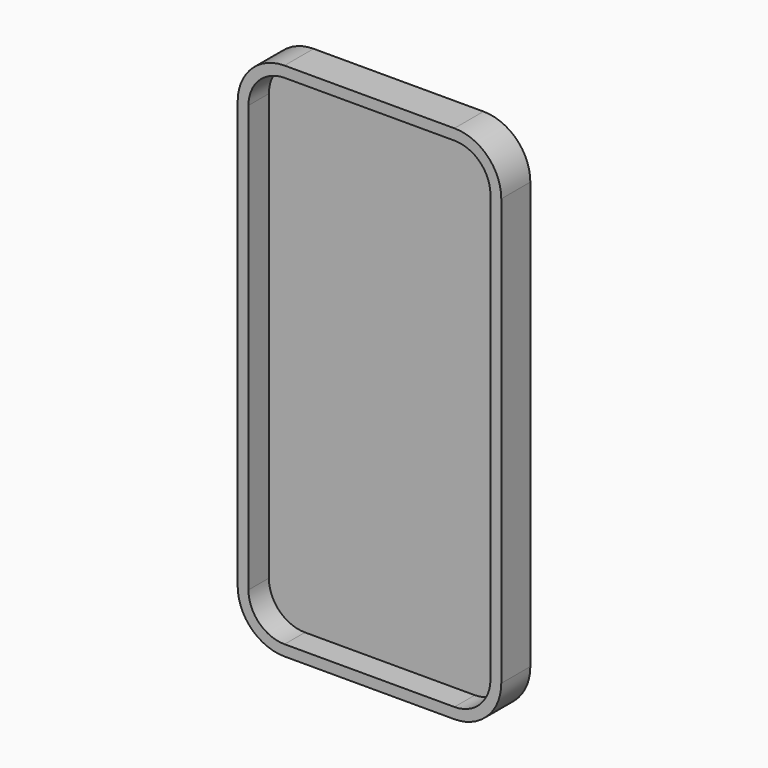
from build123d import *

# Parameters (mm, degrees)
F0_R     = 4.69
F0_W     = 58.73
F0_H     = 103.15
F0_R_2   = 2.195
F0_R_3   = 1.058193308
F0_R_4   = 5.3501775611
F1_DEPTH = 7.08
F2_DEPTH = 7.08
F4_DEPTH = 0.8
F5_T     = 3


# Not quite as in the source:
# - a feature of the source that left no trace in its solid (it failed there, or was rolled back) is left out


with BuildPart() as f1:
    # F0 (on Front) → F1 (new body)
    with BuildSketch(Plane.XZ):
        with BuildLine():
            Line((23.565, 69.16), (-23.565, 69.16))
            ThreePointArc((-23.565, 69.16), (-30.6360678119, 66.2310678119), (-33.565, 59.16))
            Line((-33.565, 59.16), (-33.565, -59.16))
            ThreePointArc((-33.565, -59.16), (-30.6360678119, -66.2310678119), (-23.565, -69.16))
            Line((-23.565, -69.16), (23.565, -69.16))
            ThreePointArc((23.565, -69.16), (30.6360678119, -66.2310678119), (33.565, -59.16))
            Line((33.565, -59.16), (33.565, 59.16))
            ThreePointArc((33.565, 59.16), (30.6360678119, 66.2310678119), (23.565, 69.16))
        make_face()
        with Locations((0, -60.0285455585)):
            Circle(F0_R, mode=Mode.SUBTRACT)
        Rectangle(F0_W, F0_H, mode=Mode.SUBTRACT)
        with Locations((10.2654388174, 59.16)):
            Circle(F0_R_2, mode=Mode.SUBTRACT)
        with Locations((14.2954164479, 59.1465724891)):
            Circle(F0_R_3, mode=Mode.SUBTRACT)
        with Locations((21.3369000703, 59.16)):
            Circle(F0_R_4, mode=Mode.SUBTRACT)
        Rectangle(F0_W, F0_H)
        with Locations((21.3369000703, 59.16)):
            Circle(F0_R_4)
        with Locations((0, -60.0285455585)):
            Circle(F0_R)
        with Locations((10.2654388174, 59.16)):
            Circle(F0_R_2)
        with Locations((14.2954164479, 59.1465724891)):
            Circle(F0_R_3)
    extrude(amount=F1_DEPTH)

    # F0 (on Front) → F2 (join)
    with BuildSketch(Plane.XZ):
        Rectangle(F0_W, F0_H)
        with Locations((0, -60.0285455585)):
            Circle(F0_R)
    extrude(amount=F2_DEPTH)

    # F0 (on Front) → F4 (join)
    with BuildSketch(Plane.XZ):
        with Locations((21.3369000703, 59.16)):
            Circle(F0_R_4)
    extrude(amount=F4_DEPTH)

    # F5
    f5_openings = [f1.faces().sort_by_distance(p)[0] for p in [
        (0, -7.08, 0),
    ]]
    offset(amount=F5_T, openings=f5_openings, kind=Kind.INTERSECTION)


solid = f1.part
